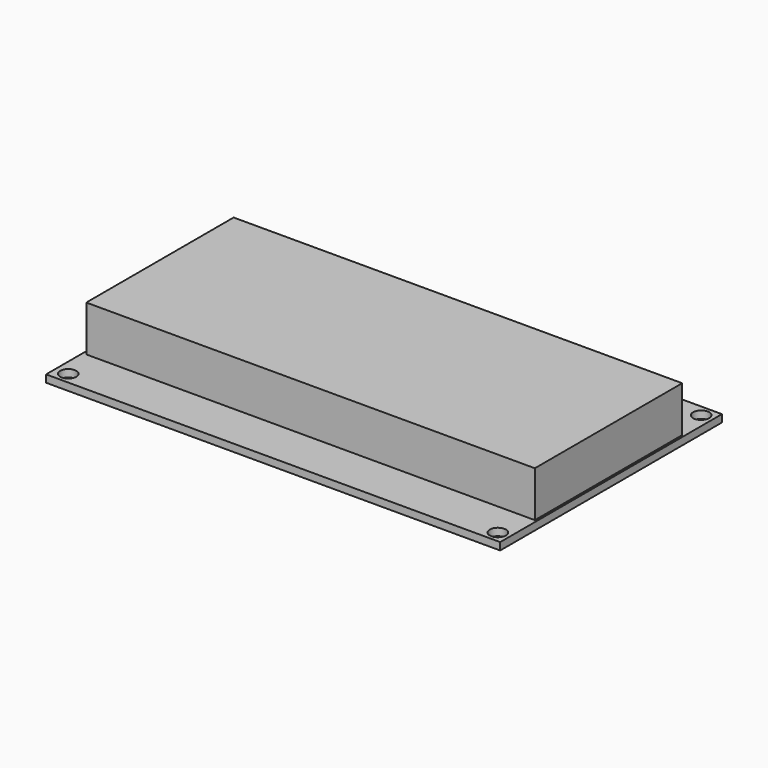
from build123d import *

# Parameters (mm, degrees)
F0_W     = 98.3
F0_H     = 60
F0_R     = 1.75
F1_DEPTH = 1.6
F2_W     = 97.1
F2_H     = 39.87
F3_DEPTH = 9.89
F4_W     = 41.93
F4_H     = 19.5
F5_DEPTH = 10.75


# Not quite as in the source:
# - a feature names something its author has since deleted; it is built from what else it names


with BuildPart() as f1:
    # F0 (on Top) → F1 (new body)
    with BuildSketch(Plane.XY):
        Rectangle(F0_W, F0_H)
        with Locations((-46.35, -27.5)):
            Circle(F0_R, mode=Mode.SUBTRACT)
        with Locations((46.65, -27.5)):
            Circle(F0_R, mode=Mode.SUBTRACT)
        with Locations((-46.35, 27.5)):
            Circle(F0_R, mode=Mode.SUBTRACT)
        with Locations((46.65, 27.5)):
            Circle(F0_R, mode=Mode.SUBTRACT)
    extrude(amount=F1_DEPTH)


with BuildPart() as f3:
    # F2 (on face) → F3 (new body)
    with BuildSketch(Plane.XY.offset(1.6)):
        with Locations((0.15, -0.125)):
            Rectangle(F2_W, F2_H)
    extrude(amount=F3_DEPTH)


with BuildPart() as f5:
    # F4 (on face) → F5 (new body)
    with BuildSketch(Plane.XY):
        with Locations((-20.385, 18.59)):
            Rectangle(F4_W, F4_H)
    extrude(amount=-F5_DEPTH)


solid = Compound([f1.part, f3.part, f5.part])
